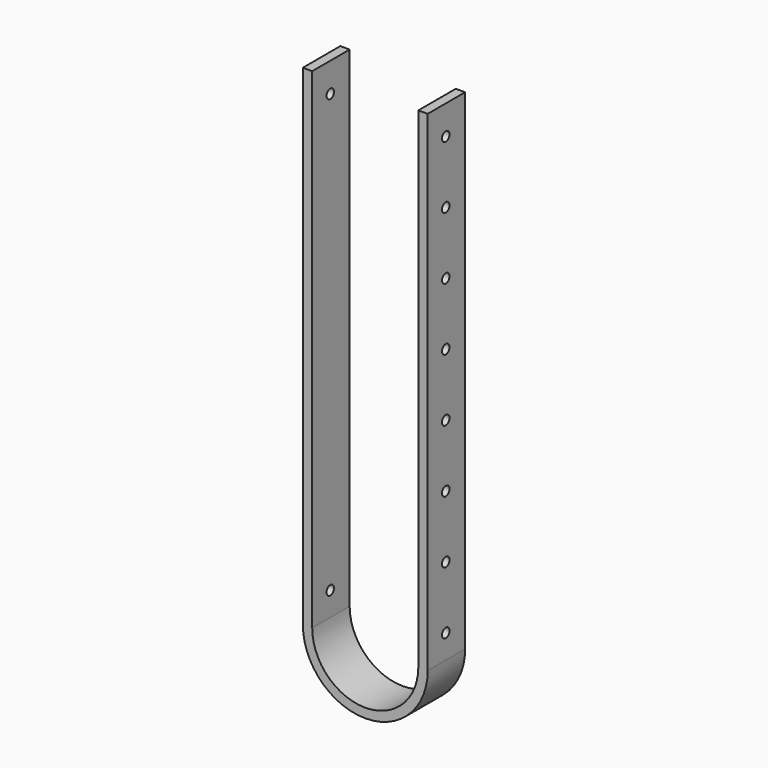
from build123d import *

# Parameters (mm, degrees)
F1_DEPTH = 15
F3_D     = 3
F3_DEPTH = 18.8319625536
F4_D     = 3


# Not quite as in the source:
# - a feature names something its author has since deleted; it is built from what else it names


with BuildPart() as f1:
    # F0 (on Front) → F1 (new body)
    with BuildSketch(Plane.XZ):
        with BuildLine():
            Line((-18.1690374464, 28.586239934), (-21.1690374464, 28.586239934))
            Line((-21.1690374464, 28.586239934), (-21.1690374464, -128.413760066))
            ThreePointArc((-21.1690374464, -128.413760066), (-1.1690374464, -148.413760066), (18.8309625536, -128.413760066))
            Line((18.8309625536, -128.413760066), (18.8309625536, 28.586239934))
            Line((18.8309625536, 28.586239934), (15.8309625536, 28.586239934))
            Line((15.8309625536, 28.586239934), (15.8309625536, -128.413760066))
            ThreePointArc((15.8309625536, -128.413760066), (-1.1690374464, -145.413760066), (-18.1690374464, -128.413760066))
            Line((-18.1690374464, -128.413760066), (-18.1690374464, 28.586239934))
        make_face()
    extrude(amount=F1_DEPTH)

    # F3 (through all, one way)
    with BuildSketch(Plane(origin=(0, 0, 0), x_dir=(0, 1, 0), z_dir=(-1, 0, 0))):
        with Locations((-7.7703874558, 0.7461506128), (-7.7703874558, 20.7461506128), (-7.7703874558, 40.7461506128), (-7.7703874558, 60.7461506128), (-7.7703874558, 80.7461506128), (-7.7703874558, 100.7461506128), (-7.7703874558, 120.7461506128), (-7.7703874558, -19.2538493872)):
            Circle(F3_D / 2)
    extrude(amount=-F3_DEPTH, mode=Mode.SUBTRACT)

    # F4 (through all)
    with Locations(Plane.YZ):
        with Locations((-7.7703874558, 19.2538493872), (-7.7703874558, -120.7461506128)):
            Hole(F4_D / 2)


solid = f1.part
